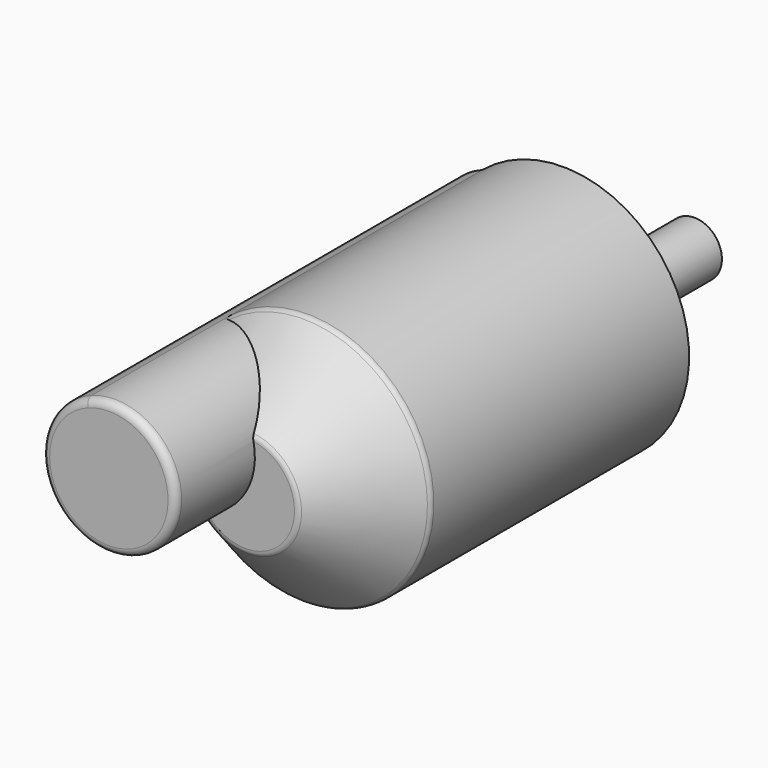
from build123d import *

# Parameters (mm, degrees)
F1_DEPTH    = 500
F0_R        = 27.8691255666
F2_DEPTH    = 400
F3_DEPTH    = 100
F4_SIZE     = 75
F5_R        = 7.62
F6_R        = 7.62
F7_T4_ANGLE = 328.4905382485
F7_S5_R     = 67.3118629199
F7_T6_DEPTH = 190


# Not quite as in the source:
# - a fillet or chamfer that OpenCascade refuses, or shapes differently, is made with other operations: its cross-section is extruded or revolved along the edge and cut away or added


with BuildPart() as f1:
    # F0 (on Front) → F1 (new body)
    with BuildSketch(Plane.XZ):
        with BuildLine():
            ThreePointArc((9.2527889353, 34.7813107073), (-19.6042711183, 90.0272610229), (-81.4330097892, 97.9045711963))
            ThreePointArc((-81.4330097892, 97.9045711963), (-109.241980875, 65.4433324256), (-124.7430483487, 25.6088272504))
            ThreePointArc((-124.7430483487, 25.6088272504), (-53.4620995229, -32.373396615), (9.2527889353, 34.7813107073))
        make_face()
        with BuildLine():
            ThreePointArc((-124.7430483487, 25.6088272504), (-109.241980875, 65.4433324256), (-81.4330097892, 97.9045711963))
            ThreePointArc((-81.4330097892, 97.9045711963), (-115.8022592462, 69.3733827123), (-124.7430483487, 25.6088272504))
        make_face()
    extrude(amount=F1_DEPTH)

    # F0 (on Front) → F2 (join)
    with BuildSketch(Plane.XZ):
        with BuildLine():
            ThreePointArc((-124.7430483487, 25.6088272504), (-12.870314303, -126.6925220927), (127.3445724971, 0))
            ThreePointArc((127.3445724971, 0), (54.0674963619, 115.2967735091), (-81.4330097892, 97.9045711963))
            ThreePointArc((-81.4330097892, 97.9045711963), (-19.6042711183, 90.0272610229), (9.2527889353, 34.7813107073))
            ThreePointArc((9.2527889353, 34.7813107073), (-53.4620995229, -32.373396615), (-124.7430483487, 25.6088272504))
        make_face()
        with Locations((52.5650605559, 30.6920967996)):
            Circle(F0_R, mode=Mode.SUBTRACT)
        with Locations((52.5650605559, 30.6920967996)):
            Circle(F0_R)
    extrude(amount=F2_DEPTH)

    # F0 (on Front) → F3 (join)
    with BuildSketch(Plane.XZ):
        with Locations((52.5650605559, 30.6920967996)):
            Circle(F0_R)
    extrude(amount=-F3_DEPTH)

    # F4
    f4_edges = [f1.edges().sort_by_distance(p)[0] for p in [
        (109.241981, -400, -65.443332),
    ]]
    chamfer(f4_edges, length=F4_SIZE)

    # F5
    f5_edges = [f1.edges().sort_by_distance(p)[0] for p in [
        (-125.370937, -500, 34.781311),
    ]]
    fillet(f5_edges, radius=F5_R)

    # F6
    f6_edges = [f1.edges().sort_by_distance(p)[0] for p in [
        (44.903561, -400, -26.900269),
    ]]
    fillet(f6_edges, radius=F6_R)

    # F7: fillet of radius 7.62 on 1 edges, made by hand


with BuildPart() as f7_tool2:
    # F7_s3 → F7_t4 (revolve)
    with BuildSketch(Plane(origin=(0, 0, 0), x_dir=(0, 1, 0), z_dir=(0.2616792898, 0, 0.9651548836))):
        with BuildLine():
            ThreePointArc((-327.2318463274, 125.1127261697), (-324.7597404093, 126.7645345348), (-321.8436926547, 127.3445724971))
            Line((-321.8436926547, 127.3445724971), (-325, 127.3445724971))
            Line((-325, 127.3445724971), (-327.2318463274, 125.1127261697))
        make_face()
    revolve(axis=Axis((0, -325, 0), (0, -1, 0)), revolution_arc=F7_T4_ANGLE)

    # F7_s5 → F7_t6 (cut, symmetric)
    with BuildSketch(Plane.XZ.offset(321.8)):
        with Locations((-58.0590739846, 34.7813107073)):
            Circle(F7_S5_R)
    extrude(amount=F7_T6_DEPTH, both=True, mode=Mode.SUBTRACT)


with BuildPart() as f1_1:
    add(f1.part)

    # F7_t1: cut F7_tool2
    add(f7_tool2.part, mode=Mode.SUBTRACT)


solid = f1_1.part
